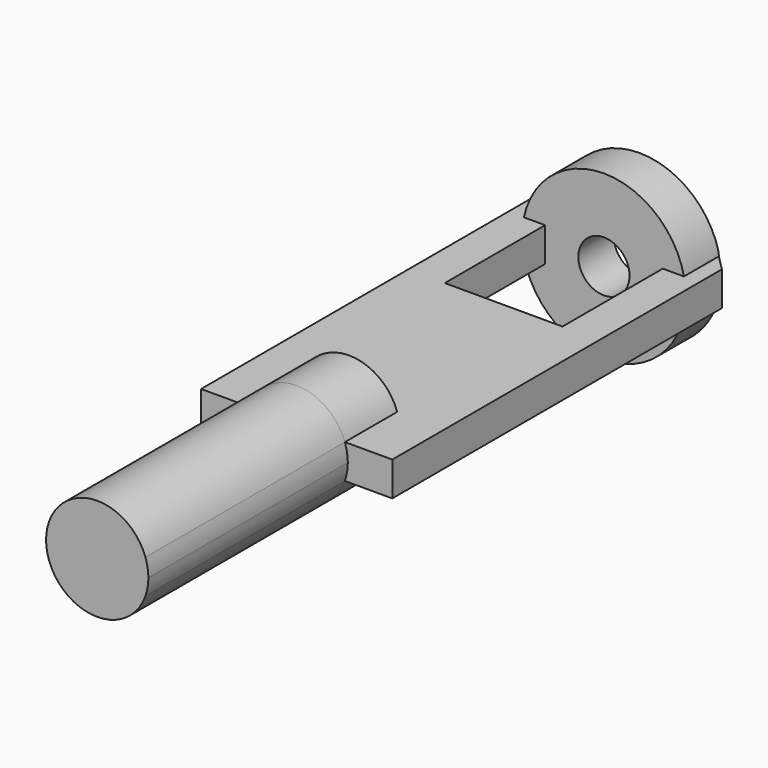
from build123d import *

# Parameters (mm, degrees)
F0_R          = 12.7
F0_R_2        = 3.96875
F1_DEPTH      = 6.8834
F3_DEPTH      = 2.6543
F4_T1_DEPTH   = 18.3727495789
F6_DEPTH      = 38.6842
F6_DEPTH_BACK = 10.16


# Not quite as in the source:
# - a fillet or chamfer that OpenCascade refuses, or shapes differently, is made with other operations: its cross-section is extruded or revolved along the edge and cut away or added


with BuildPart() as f1:
    # F0 (on Front) → F1 (new body)
    with BuildSketch(Plane.XZ):
        Circle(F0_R)
        Circle(F0_R_2, mode=Mode.SUBTRACT)
    extrude(amount=F1_DEPTH)

    # F2 (on Top) → F3 (join, symmetric)
    with BuildSketch(Plane.XY):
        Polygon((-9.1313, 0), (-14.8336, 0), (-14.8336, -66.4845), (14.8336, -66.4845), (14.8336, 0), (9.1313, 0), (9.1313, -26.3398), (-9.1313, -26.3398), align=None)
    extrude(amount=F3_DEPTH, both=True)

    # F4: chamfer of 2.54 on 2 edges, made by hand

    # F4_s2 → F4_t1 (cut)
    with BuildSketch(Plane.XY.offset(-9.1863747894)):
        Polygon((12.2936, 0), (14.8336, -2.54), (14.8336, 0), align=None)
        Polygon((-12.2936, 0), (-14.8336, -2.54), (-14.8336, 0), align=None)
    extrude(amount=F4_T1_DEPTH, mode=Mode.SUBTRACT)

    # F5 (on face) → F6 (join, two sides)
    with BuildSketch(Plane.XZ.offset(66.4845)) as f6_sk:
        with BuildLine():
            ThreePointArc((-7.4805479585, -2.6543), (0, -7.9375), (7.4805479585, -2.6543))
            Line((7.4805479585, -2.6543), (-7.4805479585, -2.6543))
        make_face()
        with BuildLine():
            ThreePointArc((7.4805479585, -2.6543), (7.8224278735, -1.3466730912), (7.9375, 0))
            ThreePointArc((7.9375, 0), (7.8224278735, 1.3466730912), (7.4805479585, 2.6543))
            Line((7.4805479585, 2.6543), (-7.4805479585, 2.6543))
            ThreePointArc((-7.4805479585, 2.6543), (-7.9375, 0), (-7.4805479585, -2.6543))
            Line((-7.4805479585, -2.6543), (7.4805479585, -2.6543))
        make_face()
        with BuildLine():
            Line((-7.4805479585, 2.6543), (7.4805479585, 2.6543))
            ThreePointArc((7.4805479585, 2.6543), (0, 7.9375), (-7.4805479585, 2.6543))
        make_face()
    extrude(amount=F6_DEPTH)
    extrude(f6_sk.sketch, amount=-F6_DEPTH_BACK)


solid = f1.part
